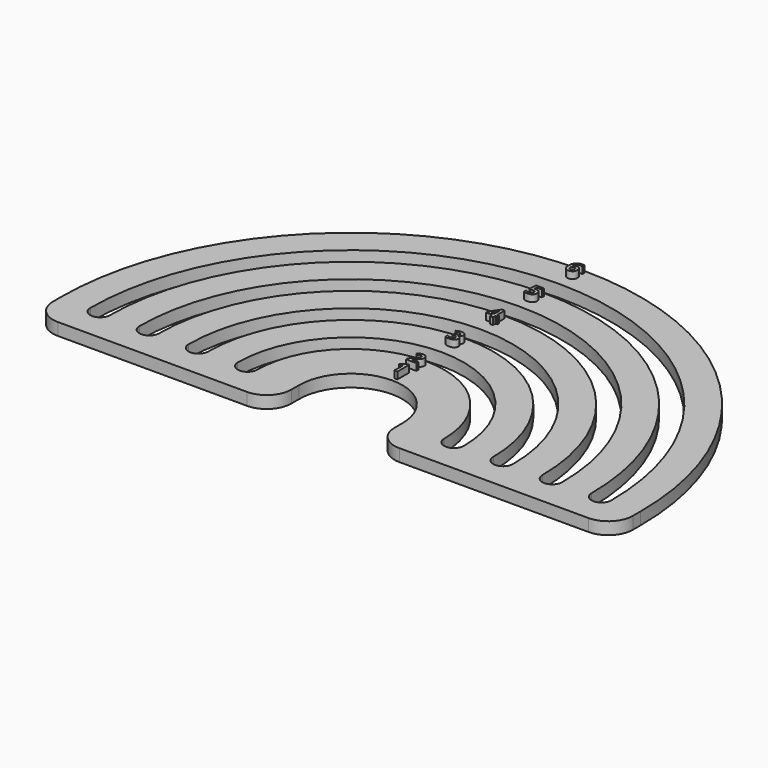
from build123d import *

# Parameters (mm, degrees)
F1_DEPTH     = 3.175
F2_R         = 6.35
F3_TEXT_SIZE = 5.2916666667
F4_DEPTH     = 1.778


# Not quite as in the source:
# - Text() gives the source's letters only with a copy of the font that has no kerning and outlines rounded to 1/6400 em; it was checked with that copy


with BuildPart() as f1:
    # F0 (on Top) → F1 (new body)
    with BuildSketch(Plane.XY):
        with BuildLine():
            Line((74.93, -8.89), (74.93, 0))
            ThreePointArc((74.93, 0), (0, 74.93), (-74.93, 0))
            Line((-74.93, 0), (-74.93, -8.89))
            Line((-74.93, -8.89), (-13.335, -8.89))
            Line((-13.335, -8.89), (-13.335, 0))
            ThreePointArc((-13.335, 0), (0, 13.335), (13.335, 0))
            Line((13.335, 0), (13.335, -8.89))
            Line((13.335, -8.89), (74.93, -8.89))
        make_face()
        with BuildLine():
            ThreePointArc((29.21, 0), (26.67, -2.54), (24.13, 0))
            ThreePointArc((24.13, 0), (0, 24.13), (-24.13, 0))
            ThreePointArc((-24.13, 0), (-26.67, -2.54), (-29.21, 0))
            ThreePointArc((-29.21, 0), (0, 29.21), (29.21, 0))
        make_face(mode=Mode.SUBTRACT)
        with BuildLine():
            ThreePointArc((41.91, 0), (39.37, -2.54), (36.83, 0))
            ThreePointArc((36.83, 0), (0, 36.83), (-36.83, 0))
            ThreePointArc((-36.83, 0), (-39.37, -2.54), (-41.91, 0))
            ThreePointArc((-41.91, 0), (0, 41.91), (41.91, 0))
        make_face(mode=Mode.SUBTRACT)
        with BuildLine():
            ThreePointArc((54.61, 0), (52.07, -2.54), (49.53, 0))
            ThreePointArc((49.53, 0), (0, 49.53), (-49.53, 0))
            ThreePointArc((-49.53, 0), (-52.07, -2.54), (-54.61, 0))
            ThreePointArc((-54.61, 0), (0, 54.61), (54.61, 0))
        make_face(mode=Mode.SUBTRACT)
        with BuildLine():
            ThreePointArc((67.31, 0), (64.77, -2.54), (62.23, 0))
            ThreePointArc((62.23, 0), (0, 62.23), (-62.23, 0))
            ThreePointArc((-62.23, 0), (-64.77, -2.54), (-67.31, 0))
            ThreePointArc((-67.31, 0), (0, 67.31), (67.31, 0))
        make_face(mode=Mode.SUBTRACT)
    extrude(amount=F1_DEPTH)

    # F2
    f2_edges = [f1.edges().sort_by_distance(p)[0] for p in [
        (-74.93, -8.89, 1.5875),
        (-13.335, -8.89, 1.5875),
        (13.335, -8.89, 1.5875),
        (74.93, -8.89, 1.5875),
    ]]
    fillet(f2_edges, radius=F2_R)

    # F3 (on face) → F4 (join)
    with BuildSketch(Plane.XY.offset(3.175)):
        with Locations((-1.5876767721, 14.3141919924)):
            Text('1', F3_TEXT_SIZE, font='Open Sans', font_style=FontStyle.BOLD, text_align=(TextAlign.LEFT, TextAlign.BOTTOM))
        with Locations((-1.5978352865, 19.6161139756)):
            Text('2', F3_TEXT_SIZE, font='Open Sans', font_style=FontStyle.BOLD, text_align=(TextAlign.LEFT, TextAlign.BOTTOM))
        with Locations((-1.563108724, 57.4264785322)):
            Text('5', F3_TEXT_SIZE, font='Open Sans', font_style=FontStyle.BOLD, text_align=(TextAlign.LEFT, TextAlign.BOTTOM))
        with Locations((-1.6404166667, 44.8934544054)):
            Text('4', F3_TEXT_SIZE, font='Open Sans', font_style=FontStyle.BOLD, text_align=(TextAlign.LEFT, TextAlign.BOTTOM))
        with Locations((-1.5796451823, 32.1567812935)):
            Text('3', F3_TEXT_SIZE, font='Open Sans', font_style=FontStyle.BOLD, text_align=(TextAlign.LEFT, TextAlign.BOTTOM))
        with Locations((-1.5978352865, 70.4099303111)):
            Text('6', F3_TEXT_SIZE, font='Open Sans', font_style=FontStyle.BOLD, text_align=(TextAlign.LEFT, TextAlign.BOTTOM))
    extrude(amount=F4_DEPTH)


solid = f1.part
